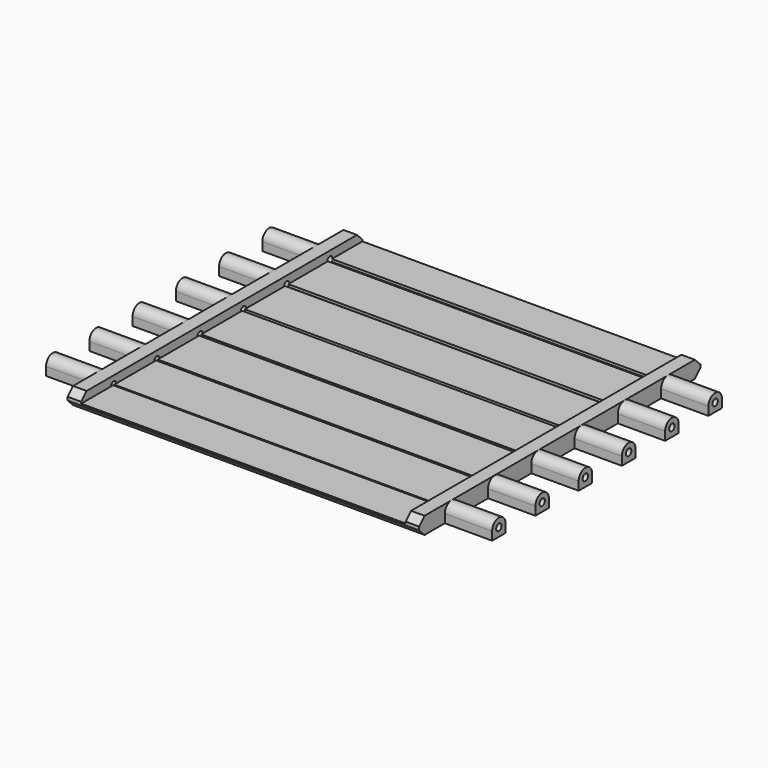
from build123d import *

# Parameters (mm, degrees)
F0_W      = 70
F0_H      = 52
F1_DEPTH  = 2.5
F2_R      = 0.5
F3_DEPTH  = 2
F5_DEPTH  = 7
F6_W      = 44
F6_H      = 52
F7_DEPTH  = 25
F10_W     = 48
F10_H     = 52
F11_DEPTH = 1.25
F12_W     = 48
F12_H     = 0.2
F12_H_2   = 0.75
F13_DEPTH = 0.375
F15_DEPTH = 60
F16_R     = 0.5
F17_DEPTH = 9
F18_R     = 0.5
F19_DEPTH = 9


# Not quite as in the source:
# - a feature names something its author has since deleted; it is built from what else it names


with BuildPart() as f1:
    # F0 (on Top) → F1 (new body)
    with BuildSketch(Plane.XY):
        with Locations((35, 26)):
            Rectangle(F0_W, F0_H)
    extrude(amount=F1_DEPTH)

    # F2 (on face) → F3 (cut)
    with BuildSketch(Plane(origin=(0, 0, 0), x_dir=(0, -1, 0), z_dir=(-1, 0, 0))):
        with Locations((-46, 1.25)):
            Circle(F2_R)
        with Locations((-38, 1.25)):
            Circle(F2_R)
        with Locations((-30, 1.25)):
            Circle(F2_R)
        with Locations((-22, 1.25)):
            Circle(F2_R)
        with Locations((-14, 1.25)):
            Circle(F2_R)
        with Locations((-6, 1.25)):
            Circle(F2_R)
    extrude(amount=-F3_DEPTH, mode=Mode.SUBTRACT)

    # F4 (on face) → F5 (join)
    with BuildSketch(Plane(origin=(0, 0, 0), x_dir=(0, -1, 0), z_dir=(-1, 0, 0))):
        with BuildLine():
            Line((-44.75, 0), (-44.75, 1.25))
            ThreePointArc((-44.75, 1.25), (-46, 2.5), (-47.25, 1.25))
            Line((-47.25, 1.25), (-47.25, 0))
            Line((-47.25, 0), (-44.75, 0))
        make_face()
        with BuildLine():
            Line((-36.75, 0), (-36.75, 1.25))
            ThreePointArc((-36.75, 1.25), (-38, 2.5), (-39.25, 1.25))
            Line((-39.25, 1.25), (-39.25, 0))
            Line((-39.25, 0), (-36.75, 0))
        make_face()
        with BuildLine():
            Line((-28.75, 0), (-28.75, 1.25))
            ThreePointArc((-28.75, 1.25), (-30, 2.5), (-31.25, 1.25))
            Line((-31.25, 1.25), (-31.25, 0))
            Line((-31.25, 0), (-28.75, 0))
        make_face()
        with BuildLine():
            Line((-20.75, 0), (-20.75, 1.25))
            ThreePointArc((-20.75, 1.25), (-22, 2.5), (-23.25, 1.25))
            Line((-23.25, 1.25), (-23.25, 0))
            Line((-23.25, 0), (-20.75, 0))
        make_face()
        with BuildLine():
            Line((-12.75, 0), (-12.75, 1.25))
            ThreePointArc((-12.75, 1.25), (-14, 2.5), (-15.25, 1.25))
            Line((-15.25, 1.25), (-15.25, 0))
            Line((-15.25, 0), (-12.75, 0))
        make_face()
        with BuildLine():
            Line((-4.75, 0), (-4.75, 1.25))
            ThreePointArc((-4.75, 1.25), (-6, 2.5), (-7.25, 1.25))
            Line((-7.25, 1.25), (-7.25, 0))
            Line((-7.25, 0), (-4.75, 0))
        make_face()
    extrude(amount=F5_DEPTH)

    # F6 (on face) → F7 (cut)
    with BuildSketch(Plane.XY.offset(2.5)):
        with Locations((48, 26)):
            Rectangle(F6_W, F6_H)
    extrude(amount=-F7_DEPTH, mode=Mode.SUBTRACT)

    # F9: F1 across plane


with BuildPart() as f1_1:
    add(f1.part)
    add(f1.part.mirror(Plane(origin=(26, 26, 1.25), x_dir=(0, 1, 0), z_dir=(1, 0, 0))))

    # F10 (on face) → F11 (cut)
    with BuildSketch(Plane.XY.offset(2.5)):
        with Locations((26, 26)):
            Rectangle(F10_W, F10_H)
    extrude(amount=-F11_DEPTH, mode=Mode.SUBTRACT)

    # F12 (on face) → F13 (cut)
    with BuildSketch(Plane.XY.offset(1.25)):
        with Locations((26, 6)):
            Rectangle(F12_W, F12_H)
        with Locations((26, 46)):
            Rectangle(F12_W, F12_H_2)
        Polygon((2, 14.15), (2, 14), (2, 13.85), (50, 13.85), (50, 14.15), align=None)
        Polygon((2, 22.2), (2, 22), (2, 21.8), (50, 21.8), (50, 22.2), align=None)
        Polygon((2, 30.25), (2, 30), (2, 29.75), (50, 29.75), (50, 30.25), align=None)
        Polygon((2, 38.3), (2, 38), (2, 37.7), (50, 37.7), (50, 38.3), align=None)
    extrude(amount=-F13_DEPTH, mode=Mode.SUBTRACT)

    # F14 (on face) → F15 (cut)
    with BuildSketch(Plane(origin=(0, 0, 0), x_dir=(0, -1, 0), z_dir=(-1, 0, 0))):
        Polygon((-51, 2.5), (-52, 2.5), (-52, 1.5), align=None)
        Polygon((-52, 1), (-52, 0), (-51, 0), align=None)
        Polygon((-1, 0), (0, 0), (0, 1), align=None)
        Polygon((0, 1.5), (0, 2.5), (-1, 2.5), align=None)
    extrude(amount=-F15_DEPTH, mode=Mode.SUBTRACT)

    # F16 (on face) → F17 (cut)
    with BuildSketch(Plane(origin=(-7, 0, 0), x_dir=(0, -1, 0), z_dir=(-1, 0, 0))):
        with Locations((-46, 1.25)):
            Circle(F16_R)
        with Locations((-38, 1.25)):
            Circle(F16_R)
        with Locations((-30, 1.25)):
            Circle(F16_R)
        with Locations((-22, 1.25)):
            Circle(F16_R)
        with Locations((-14, 1.25)):
            Circle(F16_R)
        with Locations((-6, 1.25)):
            Circle(F16_R)
    extrude(amount=-F17_DEPTH, mode=Mode.SUBTRACT)

    # F18 (on face) → F19 (cut)
    with BuildSketch(Plane.YZ.offset(59)):
        with Locations((6, 1.25)):
            Circle(F18_R)
        with Locations((14, 1.25)):
            Circle(F18_R)
        with Locations((22, 1.25)):
            Circle(F18_R)
        with Locations((30, 1.25)):
            Circle(F18_R)
        with Locations((38, 1.25)):
            Circle(F18_R)
        with Locations((46, 1.25)):
            Circle(F18_R)
    extrude(amount=-F19_DEPTH, mode=Mode.SUBTRACT)


solid = f1_1.part
